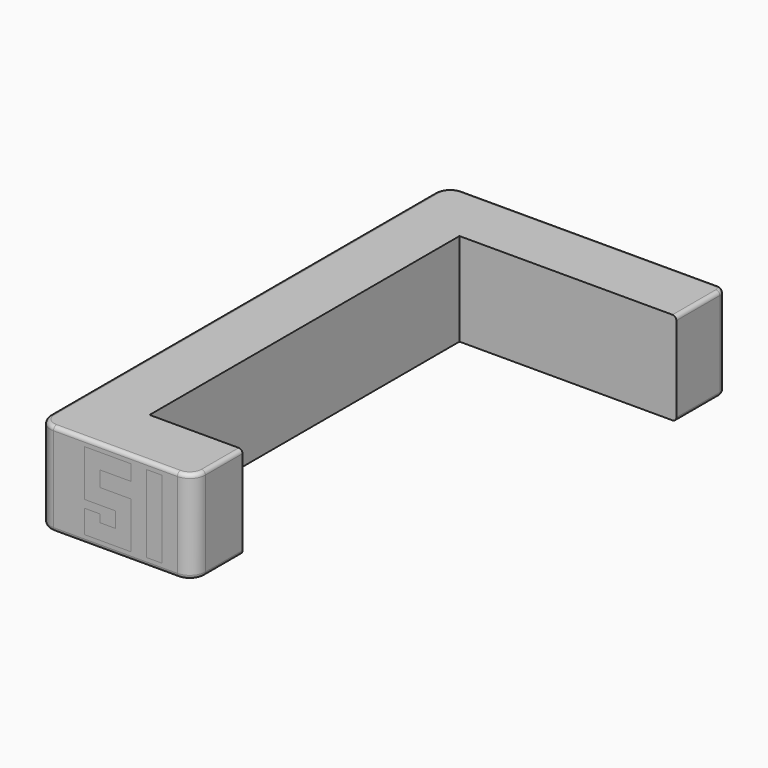
from build123d import *

# Parameters (mm, degrees)
F1_DEPTH  = 152.4
F2_R      = 25.4
F3_W      = 25.4
F3_H      = 127
F4_DEPTH  = 25.4
F5_DEPTH  = 25.4
F6_W      = 25.4
F6_H      = 127
F7_DEPTH  = 25.4
F8_DEPTH  = 25.4
F10_DEPTH = 25.4
F11_DEPTH = 25.4
F12_R     = 12.69999
F13_R     = 6.35


# Not quite as in the source:
# - a fillet or chamfer is up to 0.001 mm smaller than in the source, because OpenCascade refuses the exact size


with BuildPart() as f1:
    # F0 (on Top) → F1 (new body)
    with BuildSketch(Plane.XY):
        Polygon((355.6309728362, 708.7584971195), (-101.5690271638, 708.7584971195), (-101.5690271638, -129.4415028805), (152.4309728362, -129.4415028805), (152.4309728362, -27.8415028805), (0.0309728362, -27.8415028805), (0.0309728362, 607.1584971195), (355.6309728362, 607.1584971195), align=None)
    extrude(amount=F1_DEPTH)

    # F2
    f2_edges = [f1.edges().sort_by_distance(p)[0] for p in [
        (-101.569027, -129.441503, 76.2),
        (-101.569027, 708.758497, 76.2),
        (152.430973, -129.441503, 76.2),
    ]]
    fillet(f2_edges, radius=F2_R)

    # F3 (on face) → F4 (cut)
    with BuildSketch(Plane(origin=(-101.5690271638, 0, 0), x_dir=(0, -1, 0), z_dir=(-1, 0, 0))):
        Polygon((-384.9084971195, 114.3), (-384.9084971195, 139.7), (-461.1084971195, 139.7), (-461.1084971195, 63.5), (-410.3084971195, 63.5), (-410.3084971195, 38.1), (-435.7084971195, 38.1), (-435.7084971195, 50.8), (-461.1084971195, 50.8), (-461.1084971195, 12.7), (-384.9084971195, 12.7), (-384.9084971195, 88.9), (-435.7084971195, 88.9), (-435.7084971195, 114.3), align=None)
        with Locations((-346.8084971195, 76.2)):
            Rectangle(F3_W, F3_H)
        Polygon((-232.5084971195, 139.7), (-274.3105804205, 139.7), (-308.7084971195, 63.5), (-308.7084971195, 38.1), (-257.9084971195, 38.1), (-257.9084971195, 12.7), (-232.5084971195, 12.7), (-232.5084971195, 38.1), (-219.8084971195, 38.1), (-219.8084971195, 63.5), (-232.5084971195, 63.5), align=None)
        Polygon((-257.9084971195, 114.3), (-257.9084971195, 63.5), (-280.8404415855, 63.5), align=None, mode=Mode.SUBTRACT)
        Polygon((-118.2084971195, 114.3), (-118.2084971195, 139.7), (-194.4084971195, 139.7), (-194.4084971195, 63.5), (-143.6084971195, 63.5), (-143.6084971195, 38.1), (-169.0084971195, 38.1), (-169.0084971195, 50.8), (-194.4084971195, 50.8), (-194.4084971195, 12.7), (-118.2084971195, 12.7), (-118.2084971195, 88.9), (-169.0084971195, 88.9), (-169.0084971195, 114.3), align=None)
    extrude(amount=-F4_DEPTH, mode=Mode.SUBTRACT)


with BuildPart() as f5:
    # F5 (new): a face of the model
    f5_faces = [f1.part.faces().sort_by_distance(p)[0] for p in [
        (-76.1690271638, 424.1128449456, 74.8195652174),
    ]]
    extrude(f5_faces, amount=F5_DEPTH)


with BuildPart() as f5b:
    # F5#2 (new): a face of the model
    f5_2_faces = [f1.part.faces().sort_by_distance(p)[0] for p in [
        (-76.1690271638, 346.8084971195, 76.2),
    ]]
    extrude(f5_2_faces, amount=F5_DEPTH)


with BuildPart() as f5c:
    # F5#3 (new): a face of the model
    f5_3_faces = [f1.part.faces().sort_by_distance(p)[0] for p in [
        (-76.1690271638, 253.40953877, 138.1497674368),
    ]]
    extrude(f5_3_faces, amount=F5_DEPTH)


with BuildPart() as f5d:
    # F5#4 (new): a face of the model
    f5_4_faces = [f1.part.faces().sort_by_distance(p)[0] for p in [
        (-76.1690271638, 157.4128449456, 74.8195652174),
    ]]
    extrude(f5_4_faces, amount=F5_DEPTH)


with BuildPart() as f1_1:
    add(f1.part)

    # F6 (on face) → F7 (cut)
    with BuildSketch(Plane.XZ.offset(129.4415028805)):
        Polygon((50.8309728362, 114.3), (50.8309728362, 139.7), (-25.3690271638, 139.7), (-25.3690271638, 63.5), (25.4309728362, 63.5), (25.4309728362, 38.1), (0.0309728362, 38.1), (0.0309728362, 50.8), (-25.3690271638, 50.8), (-25.3690271638, 12.7), (50.8309728362, 12.7), (50.8309728362, 88.9), (0.0309728362, 88.9), (0.0309728362, 114.3), align=None)
        with Locations((88.9309728362, 76.2)):
            Rectangle(F6_W, F6_H)
    extrude(amount=-F7_DEPTH, mode=Mode.SUBTRACT)


with BuildPart() as f8:
    # F8 (new): a face of the model
    f8_faces = [f1_1.part.faces().sort_by_distance(p)[0] for p in [
        (11.6266250101, -104.0415028805, 74.8195652174),
    ]]
    extrude(f8_faces, amount=F8_DEPTH)


with BuildPart() as f8b:
    # F8#2 (new): a face of the model
    f8_2_faces = [f1_1.part.faces().sort_by_distance(p)[0] for p in [
        (88.9309728362, -104.0415028805, 76.2),
    ]]
    extrude(f8_2_faces, amount=F8_DEPTH)


with BuildPart() as f1_2:
    add(f1_1.part)

    # F9 (on face) → F10 (cut)
    with BuildSketch(Plane(origin=(0, 708.7584971195, 0), x_dir=(-1, 0, 0), z_dir=(0, 1, 0))):
        Polygon((-266.7309728362, 139.7), (-308.5330561372, 139.7), (-342.9309728362, 63.5), (-342.9309728362, 38.1), (-292.1309728362, 38.1), (-292.1309728362, 12.7), (-266.7309728362, 12.7), (-266.7309728362, 38.1), (-254.0309728362, 38.1), (-254.0309728362, 63.5), (-266.7309728362, 63.5), align=None)
        Polygon((-292.1309728362, 63.5), (-315.0629173021, 63.5), (-292.1309728362, 114.3), align=None, mode=Mode.SUBTRACT)
        Polygon((-152.4309728362, 114.3), (-152.4309728362, 139.7), (-228.6309728362, 139.7), (-228.6309728362, 63.5), (-177.8309728362, 63.5), (-177.8309728362, 38.1), (-203.2309728362, 38.1), (-203.2309728362, 50.8), (-228.6309728362, 50.8), (-228.6309728362, 12.7), (-152.4309728362, 12.7), (-152.4309728362, 88.9), (-203.2309728362, 88.9), (-203.2309728362, 114.3), align=None)
    extrude(amount=-F10_DEPTH, mode=Mode.SUBTRACT)


with BuildPart() as f11:
    # F11 (new): a face of the model
    f11_faces = [f1_2.part.faces().sort_by_distance(p)[0] for p in [
        (287.6320144867, 683.3584971195, 138.1497674368),
    ]]
    extrude(f11_faces, amount=F11_DEPTH)


with BuildPart() as f11b:
    # F11#2 (new): a face of the model
    f11_2_faces = [f1_2.part.faces().sort_by_distance(p)[0] for p in [
        (191.6353206623, 683.3584971195, 74.8195652174),
    ]]
    extrude(f11_2_faces, amount=F11_DEPTH)


with BuildPart() as f1_3:
    add(f1_2.part)

    # F12 (radius 12.7 in the source; OpenCascade refuses exactly that, so slightly less here)
    f12_edges = [f1_3.edges().sort_by_distance(p)[0] for p in [
        (355.630973, 708.758497, 76.2),
    ]]
    fillet(f12_edges, radius=F12_R)

    # F13
    f13_edges = [f1_3.edges().sort_by_distance(p)[0] for p in [
        (-101.569027, 289.658497, 152.4),
        (-101.569027, 289.658497, 0),
    ]]
    fillet(f13_edges, radius=F13_R)


solid = Compound([f5.part, f5b.part, f5c.part, f5d.part, f8.part, f8b.part, f11.part, f11b.part, f1_3.part])
